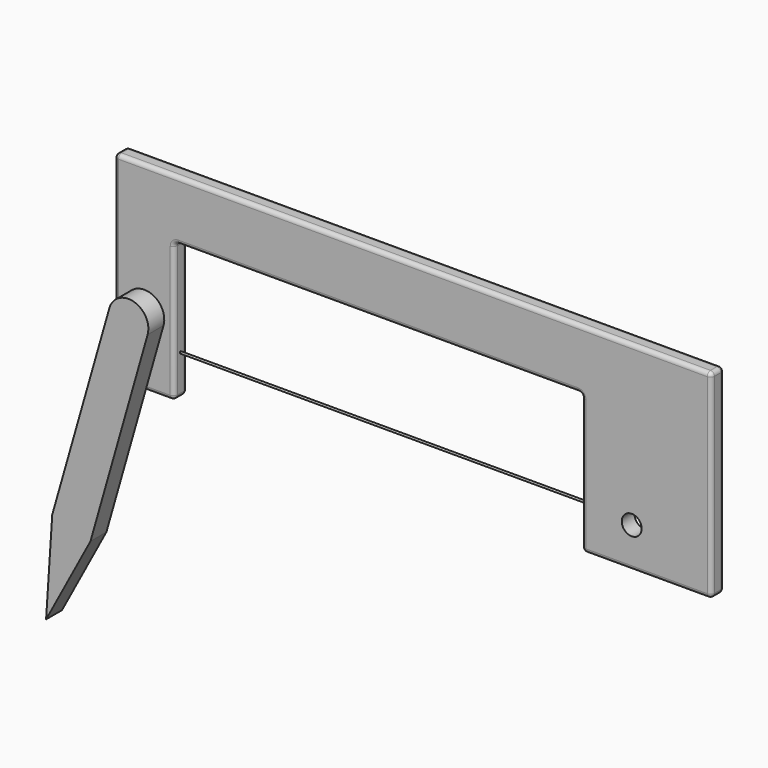
from build123d import *

# Parameters (mm, degrees)
F0_R     = 5
F1_DEPTH = 8
F2_R     = 2
F3_R     = 0.5
F4_DEPTH = 205
F6_DEPTH = 10


with BuildPart() as f1:
    # F0 (on Front) → F1 (new body)
    with BuildSketch(Plane.XZ):
        Polygon((-25, 50), (-25, -20), (40, -20), (40, 80), (-260, 80), (-260, -20), (-230, -20), (-230, 50), align=None)
        Circle(F0_R, mode=Mode.SUBTRACT)
    extrude(amount=F1_DEPTH)

    # F2
    f2_edges = [f1.edges().sort_by_distance(p)[0] for p in [
        (-260, -8, 30),
        (-245, -8, -20),
        (-230, -8, 15),
        (-127.5, -8, 50),
        (-25, -8, 15),
        (7.5, -8, -20),
        (40, -8, 30),
        (-110, -8, 80),
        (-260, -4, 80),
        (-260, -4, -20),
        (40, -4, 80),
        (40, -4, -20),
        (-25, -4, -20),
        (-25, -4, 50),
        (-230, -4, 50),
        (-230, -4, -20),
        (-245, 0, -20),
        (-230, 0, 15),
        (-127.5, 0, 50),
        (7.5, 0, -20),
        (40, 0, 30),
        (-110, 0, 80),
        (-260, 0, 30),
        (-25, 0, 15),
    ]]
    fillet(f2_edges, radius=F2_R)

    # F3 (on face) → F4 (join, through all)
    with BuildSketch(Plane(origin=(-25, 0, 0), x_dir=(0, -1, 0), z_dir=(-1, 0, 0))):
        with Locations((4, 0)):
            Circle(F3_R)
    extrude(amount=F4_DEPTH)

    # F5 (on face) → F6 (join)
    with BuildSketch(Plane.XZ.offset(8)):
        with BuildLine():
            ThreePointArc((-235.3830339919, 11.7465816491), (-242.2588387865, 24.1047088707), (-254.6169660081, 17.2289040761))
            Line((-254.6169660081, 17.2289040761), (-283.3303219183, -83.5077349835))
            Line((-283.3303219183, -83.5077349835), (-286.420911747, -130.8315102833))
            Line((-286.420911747, -130.8315102833), (-264.096389902, -88.9900574105))
            Line((-264.096389902, -88.9900574105), (-235.3830339919, 11.7465816491))
        make_face()
    extrude(amount=F6_DEPTH)


solid = f1.part
